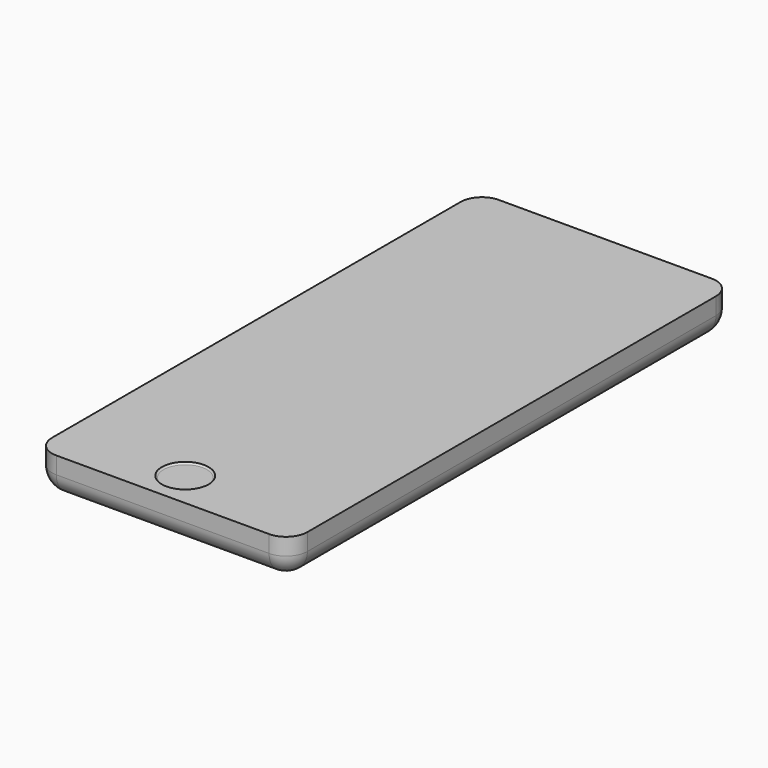
from build123d import *

# Parameters (mm, degrees)
F0_W     = 60
F0_H     = 130
F1_DEPTH = 9
F2_R     = 5
F3_R     = 5
F4_R     = 5
F5_R     = 5
F6_R     = 5.5
F7_DEPTH = 0.4
F8_R     = 0.39999


# Not quite as in the source:
# - a fillet or chamfer is up to 0.001 mm smaller than in the source, because OpenCascade refuses the exact size


with BuildPart() as f1:
    # F0 (on Top) → F1 (new body)
    with BuildSketch(Plane.XY):
        with Locations((-13.6178402903, -1.0656192899)):
            Rectangle(F0_W, F0_H)
    extrude(amount=F1_DEPTH)

    # F2
    f2_edges = [f1.edges().sort_by_distance(p)[0] for p in [
        (16.38216, -1.065619, 0),
    ]]
    fillet(f2_edges, radius=F2_R)

    # F3
    f3_edges = [f1.edges().sort_by_distance(p)[0] for p in [
        (-43.61784, -1.065619, 0),
    ]]
    fillet(f3_edges, radius=F3_R)

    # F4
    f4_edges = [f1.edges().sort_by_distance(p)[0] for p in [
        (-13.61784, 63.934381, 0),
    ]]
    fillet(f4_edges, radius=F4_R)

    # F5
    f5_edges = [f1.edges().sort_by_distance(p)[0] for p in [
        (-13.61784, -66.065619, 0),
    ]]
    fillet(f5_edges, radius=F5_R)

    # F6 (on face) → F7 (cut)
    with BuildSketch(Plane.XY.offset(9)):
        with Locations((-15.1178402903, -57.5656192899)):
            Circle(F6_R)
    extrude(amount=-F7_DEPTH, mode=Mode.SUBTRACT)

    # F8 (radius 0.4 in the source; OpenCascade refuses exactly that, so slightly less here)
    f8_edges = [f1.edges().sort_by_distance(p)[0] for p in [
        (-20.61784, -57.565619, 8.6),
    ]]
    fillet(f8_edges, radius=F8_R)


solid = f1.part
